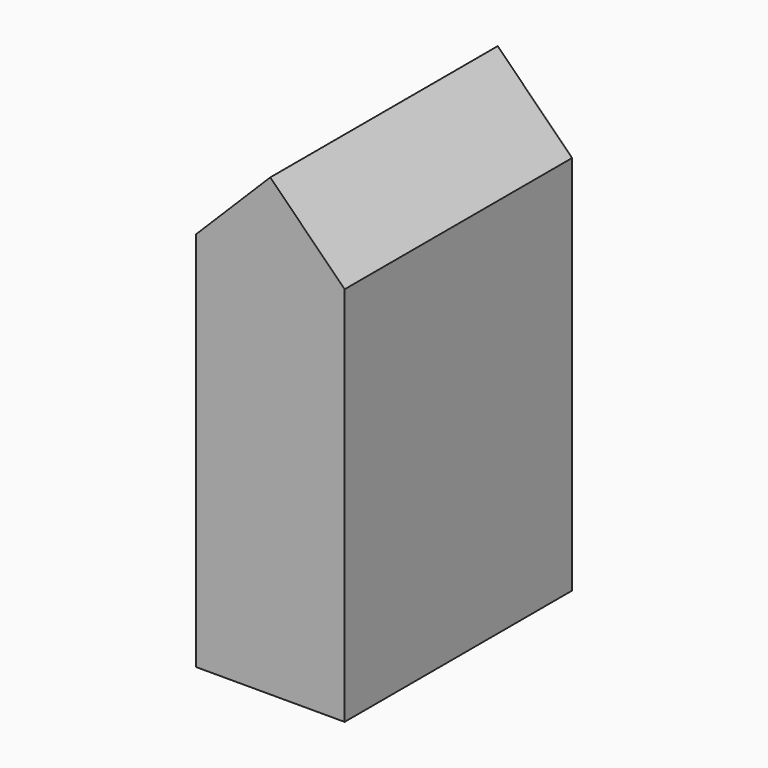
from build123d import *

# Parameters (mm, degrees)
F0_W        = 43.0329442024
F0_H        = 82.2901595384
F1_DEPTH    = 135.636
F2_T1_DEPTH = 212.9316553271
F3_W        = 19.7290945798
F3_H        = 38.1281389855
F3_R        = 12.2243381544
F3_R_2      = 14.5784118216
F3_R_3      = 9.3761022788
F4_DEPTH    = 9.652


# Not quite as in the source:
# - a fillet or chamfer that OpenCascade refuses, or shapes differently, is made with other operations: its cross-section is extruded or revolved along the edge and cut away or added


with BuildPart() as f1:
    # F0 (on Top) → F1 (new body)
    with BuildSketch(Plane.XY):
        with Locations((-110.2483123541, 24.9322196469)):
            Rectangle(F0_W, F0_H)
    extrude(amount=F1_DEPTH)

    # F2: chamfer of 25.4 on 2 edges, made by hand

    # F2_s2 → F2_t1 (cut)
    with BuildSketch(Plane.XZ.offset(-131.3980473104)):
        Polygon((-131.7647844553, 110.236), (-106.3647844553, 135.636), (-131.7647844553, 135.636), align=None)
        Polygon((-88.7318402529, 110.236), (-114.1318402529, 135.636), (-88.7318402529, 135.636), align=None)
    extrude(amount=F2_T1_DEPTH, mode=Mode.SUBTRACT)

    # F3 (on face) → F4 (cut)
    with BuildSketch(Plane(origin=(-131.7647844553, 0, 0), x_dir=(0, -1, 0), z_dir=(-1, 0, 0))):
        with Locations((-38.9040028676, 23.8969207276)):
            Rectangle(F3_W, F3_H)
        with Locations((-51.650326699, 87.2960314155)):
            Circle(F3_R)
        with Locations((-8.8670095429, 87.961062789)):
            Circle(F3_R_2)
        with Locations((-3.9901542477, 25.8919987828)):
            Circle(F3_R_3)
    extrude(amount=-F4_DEPTH, mode=Mode.SUBTRACT)


solid = f1.part
